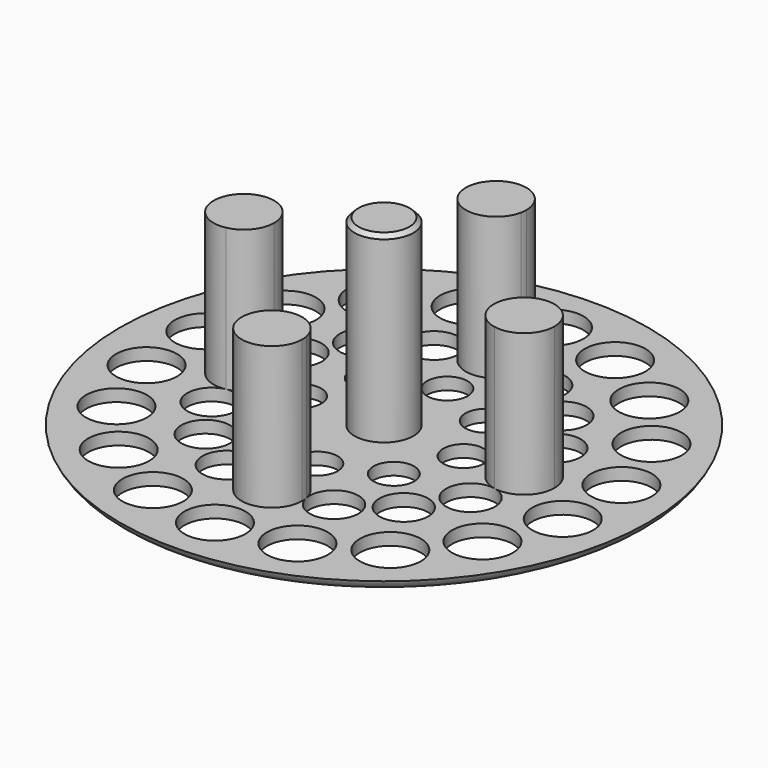
from build123d import *

# Parameters (mm, degrees)
F0_R     = 65
F0_R_2   = 7.5
F0_R_3   = 6
F0_R_4   = 5
F1_DEPTH = 3
F2_R     = 7.25
F3_DEPTH = 45
F4_SIZE  = 1
F5_R     = 6
F6_DEPTH = 35
F7_DEPTH = 3


# Not quite as in the source:
# - a fillet or chamfer that OpenCascade refuses, or shapes differently, is made with other operations: its cross-section is extruded or revolved along the edge and cut away or added


with BuildPart() as f1:
    # F0 (on Top) → F1 (new body)
    with BuildSketch(Plane.XY):
        Circle(F0_R)
        with Locations((-33.4249557037, -39.8343110422)):
            Circle(F0_R_2, mode=Mode.SUBTRACT)
        with Locations((-17.7850474529, -48.8640162809)):
            Circle(F0_R_2, mode=Mode.SUBTRACT)
        with Locations((-45.0333209968, -26)):
            Circle(F0_R_2, mode=Mode.SUBTRACT)
        with Locations((-51.2100031566, -9.0297052387)):
            Circle(F0_R_2, mode=Mode.SUBTRACT)
        with Locations((-24.3809636253, -24.3809636253)):
            Circle(F0_R_3, mode=Mode.SUBTRACT)
        with Locations((-13.1948824318, -31.8552641208)):
            Circle(F0_R_3, mode=Mode.SUBTRACT)
        with Locations((-31.8552641208, -13.1948824318)):
            Circle(F0_R_3, mode=Mode.SUBTRACT)
        with Locations((-20, -0.5201105773)):
            Circle(F0_R_4, mode=Mode.SUBTRACT)
        with Locations((-14.1421356237, -14.6622462011)):
            Circle(F0_R_4, mode=Mode.SUBTRACT)
        with Locations((0, -52)):
            Circle(F0_R_2, mode=Mode.SUBTRACT)
        with Locations((17.7850474529, -48.8640162809)):
            Circle(F0_R_2, mode=Mode.SUBTRACT)
        with Locations((0, -34.4798894227)):
            Circle(F0_R_3, mode=Mode.SUBTRACT)
        with Locations((33.4249557037, -39.8343110422)):
            Circle(F0_R_2, mode=Mode.SUBTRACT)
        with Locations((13.1948824318, -31.8552641208)):
            Circle(F0_R_3, mode=Mode.SUBTRACT)
        with Locations((0, -20.5201105773)):
            Circle(F0_R_4, mode=Mode.SUBTRACT)
        with Locations((24.3809636253, -24.3809636253)):
            Circle(F0_R_3, mode=Mode.SUBTRACT)
        with Locations((14.1421356237, -14.6622462011)):
            Circle(F0_R_4, mode=Mode.SUBTRACT)
        with Locations((31.8552641208, -13.1948824318)):
            Circle(F0_R_3, mode=Mode.SUBTRACT)
        with Locations((20, -0.5201105773)):
            Circle(F0_R_4, mode=Mode.SUBTRACT)
        with Locations((45.0333209968, -26)):
            Circle(F0_R_2, mode=Mode.SUBTRACT)
        with Locations((51.2100031566, -9.0297052387)):
            Circle(F0_R_2, mode=Mode.SUBTRACT)
        with Locations((-51.2100031566, 9.0297052387)):
            Circle(F0_R_2, mode=Mode.SUBTRACT)
        with Locations((-34.4798894227, 0)):
            Circle(F0_R_3, mode=Mode.SUBTRACT)
        with Locations((-45.0333209968, 26)):
            Circle(F0_R_2, mode=Mode.SUBTRACT)
        with Locations((-31.8552641208, 13.1948824318)):
            Circle(F0_R_3, mode=Mode.SUBTRACT)
        with Locations((-14.1421356237, 13.6220250464)):
            Circle(F0_R_4, mode=Mode.SUBTRACT)
        with Locations((-24.3809636253, 24.3809636253)):
            Circle(F0_R_3, mode=Mode.SUBTRACT)
        with Locations((-13.1948824318, 31.8552641208)):
            Circle(F0_R_3, mode=Mode.SUBTRACT)
        with Locations((-33.4249557037, 39.8343110422)):
            Circle(F0_R_2, mode=Mode.SUBTRACT)
        with Locations((-17.7850474529, 48.8640162809)):
            Circle(F0_R_2, mode=Mode.SUBTRACT)
        with Locations((14.1421356237, 13.6220250464)):
            Circle(F0_R_4, mode=Mode.SUBTRACT)
        with Locations((31.8552641208, 13.1948824318)):
            Circle(F0_R_3, mode=Mode.SUBTRACT)
        with Locations((0, 19.4798894227)):
            Circle(F0_R_4, mode=Mode.SUBTRACT)
        with Locations((13.1948824318, 31.8552641208)):
            Circle(F0_R_3, mode=Mode.SUBTRACT)
        with Locations((24.3809636253, 24.3809636253)):
            Circle(F0_R_3, mode=Mode.SUBTRACT)
        with Locations((34.4798894227, 0)):
            Circle(F0_R_3, mode=Mode.SUBTRACT)
        with Locations((51.2100031566, 9.0297052387)):
            Circle(F0_R_2, mode=Mode.SUBTRACT)
        with Locations((45.0333209968, 26)):
            Circle(F0_R_2, mode=Mode.SUBTRACT)
        with Locations((0, 34.4798894227)):
            Circle(F0_R_3, mode=Mode.SUBTRACT)
        with Locations((0, 52)):
            Circle(F0_R_2, mode=Mode.SUBTRACT)
        with Locations((17.7850474529, 48.8640162809)):
            Circle(F0_R_2, mode=Mode.SUBTRACT)
        with Locations((33.4249557037, 39.8343110422)):
            Circle(F0_R_2, mode=Mode.SUBTRACT)
    extrude(amount=F1_DEPTH)

    # F2 (on face) → F3 (join)
    with BuildSketch(Plane.XY.offset(3)):
        Circle(F2_R)
    extrude(amount=F3_DEPTH)

    # F4
    f4_edges = [f1.edges().sort_by_distance(p)[0] for p in [
        (-7.25, 0, 48),
    ]]
    chamfer(f4_edges, length=F4_SIZE)

    # F5 (on face) → F6 (join)
    with BuildSketch(Plane.XY.offset(3)):
        with BuildLine():
            ThreePointArc((7.3101707312, 33.0258059616), (7.4174953683, 33.7493298476), (7.4533854611, 34.4798894227))
            ThreePointArc((7.4533854611, 34.4798894227), (-0.7305597159, 41.8973847771), (-7.310170676, 33.0258056838))
            ThreePointArc((-7.310170676, 33.0258056838), (1.416e-07, 27.0265039616), (7.3101707312, 33.0258059616))
        make_face()
        with Locations((0, 34.4798894227)):
            Circle(F5_R, mode=Mode.SUBTRACT)
        with BuildLine():
            ThreePointArc((-33.0258056652, -7.3101706723), (-28.7183444229, -4.728377528), (-27.0265039616, 0))
            ThreePointArc((-27.0265039616, 0), (-28.7183444392, 4.7283775479), (-33.0258057157, 7.3101706823))
            ThreePointArc((-33.0258057157, 7.3101706823), (-41.9332748837, -2.58e-08), (-33.0258056652, -7.3101706723))
        make_face()
        with Locations((-34.4798894227, 0)):
            Circle(F5_R, mode=Mode.SUBTRACT)
        with BuildLine():
            ThreePointArc((-7.310170682, -33.025805714), (-0.7305597006, -41.8973847786), (7.4533854611, -34.4798894227))
            ThreePointArc((7.4533854611, -34.4798894227), (7.4174953531, -33.7493296936), (7.3101706709, -33.0258056581))
            ThreePointArc((7.3101706709, -33.0258056581), (-2.85e-08, -27.0265039616), (-7.310170682, -33.025805714))
        make_face()
        with Locations((0, -34.4798894227)):
            Circle(F5_R, mode=Mode.SUBTRACT)
        with BuildLine():
            ThreePointArc((33.0258061581, -7.3101707703), (39.2082671449, -5.7615448403), (41.9332748837, 0))
            ThreePointArc((41.9332748837, 0), (39.208266979, 5.7615449765), (33.0258057371, 7.3101706866))
            ThreePointArc((33.0258057371, 7.3101706866), (27.0265039616, -2.146e-07), (33.0258061581, -7.3101707703))
        make_face()
        with Locations((34.4798894227, 0)):
            Circle(F5_R, mode=Mode.SUBTRACT)
        with Locations((-34.4798894227, 0)):
            Circle(F5_R)
        with Locations((0, -34.4798894227)):
            Circle(F5_R)
        with Locations((34.4798894227, 0)):
            Circle(F5_R)
        with Locations((0, 34.4798894227)):
            Circle(F5_R)
    extrude(amount=F6_DEPTH)

    # F7 (add, through all): faces of the model
    f7_faces = [f1.faces().sort_by_distance(p)[0] for p in [
        (-34.4798894227, 0, 3),
        (0, -34.4798894227, 3),
        (34.4798894227, 0, 3),
        (0, 34.4798894227, 3),
    ]]
    extrude(f7_faces, amount=F7_DEPTH)

    # F8: fillet of radius 5 on 1 edges, made by hand

    # F8_s1 → F8_t2 (revolve, cut)
    with BuildSketch(Plane.XZ):
        with BuildLine():
            ThreePointArc((65, 3), (63.1560370926, 0.8166998673), (60.417424305, 0))
            Line((60.417424305, 0), (65, 0))
            Line((65, 0), (65, 3))
        make_face()
    revolve(axis=Axis((0, 0, 0), (0, 0, 1)), mode=Mode.SUBTRACT)


solid = f1.part
